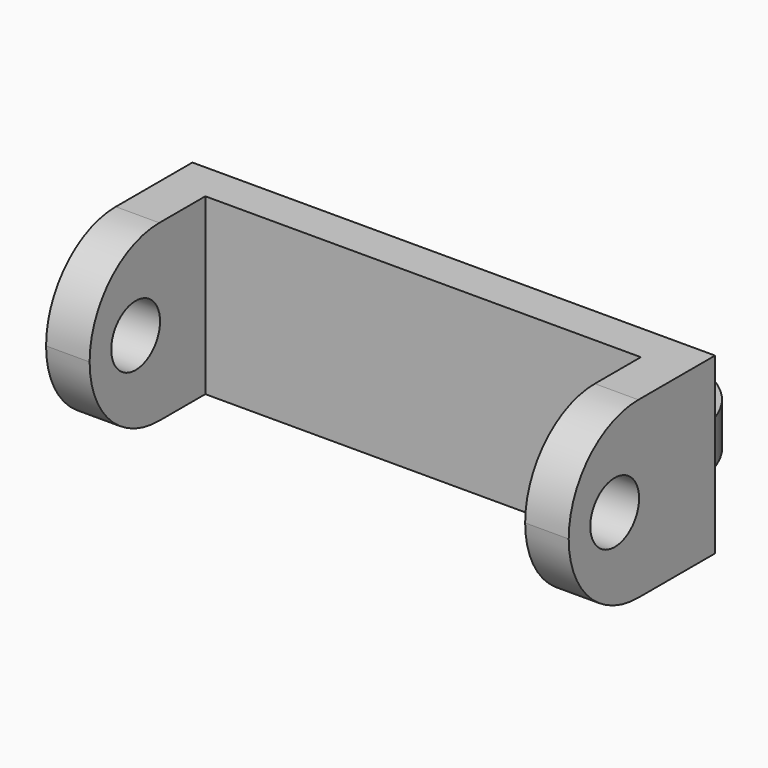
from build123d import *

# Parameters (mm, degrees)
F0_W      = 25
F0_H      = 10
F1_DEPTH  = 2.2
F0_W_2    = 2.5
F2_DEPTH  = 10.5
F3_R      = 4.99999
F4_R      = 1.75
F5_DEPTH  = 35
F6_W      = 20
F6_H      = 2.5
F7_DEPTH  = 10
F8_R      = 5
F9_R      = 1.5
F10_DEPTH = 25


# Not quite as in the source:
# - a fillet or chamfer is up to 0.001 mm smaller than in the source, because OpenCascade refuses the exact size


with BuildPart() as f1:
    # F0 (on Front) → F1 (new body)
    with BuildSketch(Plane.XZ):
        Rectangle(F0_W, F0_H)
    extrude(amount=F1_DEPTH)

    # F0 (on Front) → F2 (join)
    with BuildSketch(Plane.XZ):
        with Locations((-13.75, 0)):
            Rectangle(F0_W_2, F0_H)
        with Locations((13.75, 0)):
            Rectangle(F0_W_2, F0_H)
    extrude(amount=F2_DEPTH)

    # F3 (radius 5 in the source; OpenCascade refuses exactly that, so slightly less here)
    f3_edges = [f1.edges().sort_by_distance(p)[0] for p in [
        (13.75, -10.5, 5),
        (13.75, -10.5, -5),
        (-13.75, -10.5, -5),
        (-13.75, -10.5, 5),
    ]]
    fillet(f3_edges, radius=F3_R)

    # F4 (on face) → F5 (cut)
    with BuildSketch(Plane.YZ.offset(15)):
        with Locations((-7.2, 0)):
            Circle(F4_R)
    extrude(amount=-F5_DEPTH, mode=Mode.SUBTRACT)

    # F6 (on face) → F7 (join)
    with BuildSketch(Plane(origin=(0, 0, 0), x_dir=(-1, 0, 0), z_dir=(0, 1, 0))):
        with Locations((0, -3.75)):
            Rectangle(F6_W, F6_H)
    extrude(amount=F7_DEPTH)

    # F8
    f8_edges = [f1.edges().sort_by_distance(p)[0] for p in [
        (10, 10, -3.75),
        (-10, 10, -3.75),
    ]]
    fillet(f8_edges, radius=F8_R)

    # F9 (on face) → F10 (cut)
    with BuildSketch(Plane(origin=(0, 0, -5), x_dir=(1, 0, 0), z_dir=(0, 0, -1))):
        with Locations((0, -7.5)):
            Circle(F9_R)
    extrude(amount=-F10_DEPTH, mode=Mode.SUBTRACT)


solid = f1.part
